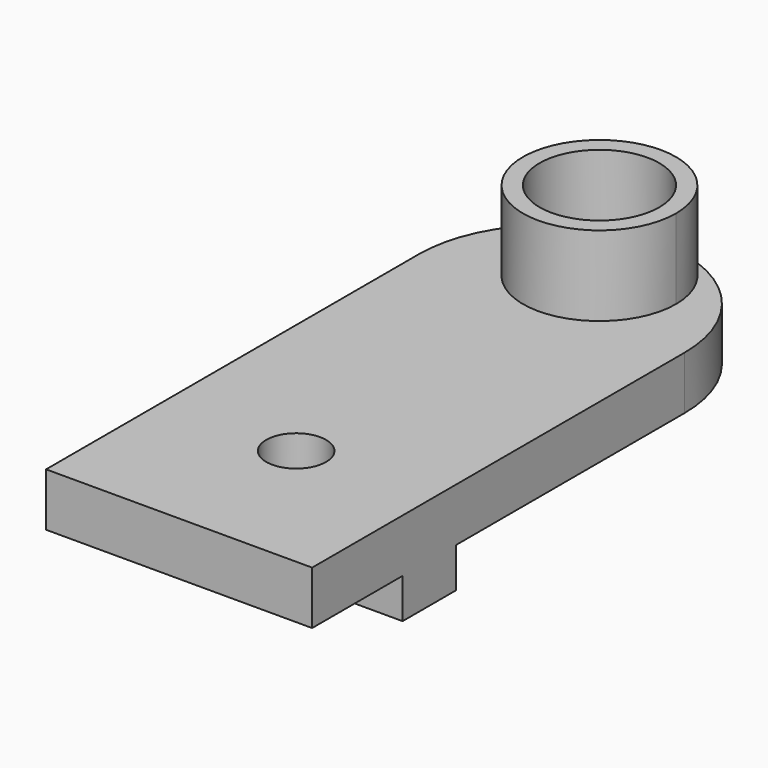
from build123d import *

# Parameters (mm, degrees)
F0_R     = 2.25
F0_R_2   = 4.5
F1_DEPTH = 4
F2_W     = 3.75
F2_H     = 5
F3_DEPTH = 3
F4_R     = 4.5
F5_DEPTH = 10


with BuildPart() as f1:
    # F0 (on Top) → F1 (new body)
    with BuildSketch(Plane.XY):
        with BuildLine():
            Line((-10, 35), (-10, 0))
            Line((-10, 0), (10, 0))
            Line((10, 0), (10, 35))
            ThreePointArc((10, 35), (0, 45), (-10, 35))
        make_face()
        with Locations((0, 11)):
            Circle(F0_R, mode=Mode.SUBTRACT)
        with Locations((0, 39.5)):
            Circle(F0_R_2, mode=Mode.SUBTRACT)
    extrude(amount=F1_DEPTH)

    # F2 (on Top) → F3 (join)
    with BuildSketch(Plane.XY):
        with Locations((-8.125, 11)):
            Rectangle(F2_W, F2_H)
        with Locations((8.125, 11)):
            Rectangle(F2_W, F2_H)
    extrude(amount=-F3_DEPTH)

    # F4 (on face) → F5 (join)
    with BuildSketch(Plane(origin=(0, 0, 0), x_dir=(1, 0, 0), z_dir=(0, 0, -1))):
        with BuildLine():
            ThreePointArc((2.4862908139, -44.6859877136), (4.8669921435, -42.5640656083), (5.7511834067, -39.5))
            ThreePointArc((5.7511834067, -39.5), (-3.0640656083, -34.6330078565), (-2.4862908139, -44.6859877136))
            ThreePointArc((-2.4862908139, -44.6859877136), (0, -45), (2.4862908139, -44.6859877136))
        make_face()
        with Locations((0, -39.5)):
            Circle(F4_R, mode=Mode.SUBTRACT)
        with BuildLine():
            ThreePointArc((2.4862908139, -44.6859877136), (0, -45), (-2.4862908139, -44.6859877136))
            ThreePointArc((-2.4862908139, -44.6859877136), (0, -45.2511834067), (2.4862908139, -44.6859877136))
        make_face()
    extrude(amount=-F5_DEPTH)


solid = f1.part
